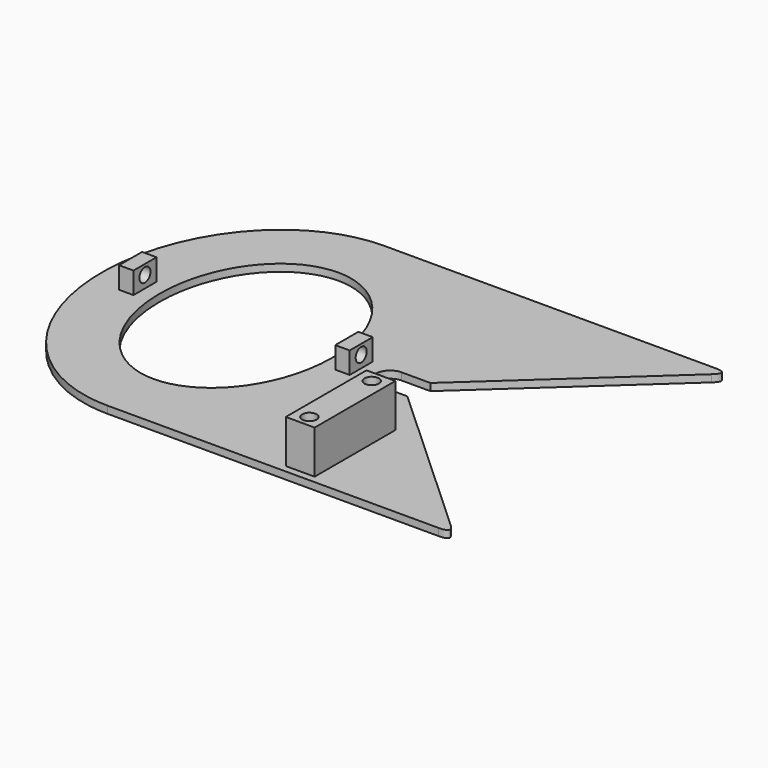
from build123d import *

# Parameters (mm, degrees)
F0_W        = 6.35
F0_H        = 12.7
F1_DEPTH    = 3.175
F3_T1_DEPTH = 35.8241837791
F4_DEPTH    = 12.7
F6_D        = 6.10108
F7_W        = 12.7
F7_H        = 44.45
F8_DEPTH    = 19.05
F9_R        = 3.175
F10_DEPTH   = 17.78
F11_DEPTH   = 17.78


# Not quite as in the source:
# - a fillet or chamfer that OpenCascade refuses, or shapes differently, is made with other operations: its cross-section is extruded or revolved along the edge and cut away or added
# - a feature of the source that left no trace in its solid (it failed there, or was rolled back) is left out


with BuildPart() as f1:
    # F0 (on Top) → F1 (new body)
    with BuildSketch(Plane.XY):
        with BuildLine():
            Line((76.2, 76.2), (-76.2, 76.2))
            add(Edge.make_bspline(
                [(-76.2, 76.2), (-139.7, 76.2), (-139.7, 0), (-139.7, -76.2), (-76.2, -76.2)],
                knots=[0, 0, 0, 1.5707963268, 1.5707963268, 3.1415926536, 3.1415926536, 3.1415926536], degree=2, weights=[1, 0.7071067812, 1, 0.7071067812, 1]))
            Line((-76.2, -76.2), (76.2, -76.2))
            Line((76.2, -76.2), (0, -6.35))
            Line((0, -6.35), (-12.7, -6.35))
            ThreePointArc((-12.7, -6.35), (-19.05, 0), (-12.7, 6.35))
            Line((-12.7, 6.35), (0, 6.35))
            Line((0, 6.35), (76.2, 76.2))
        make_face()
        with Locations((-123.825, 0)):
            Rectangle(F0_W, F0_H, mode=Mode.SUBTRACT)
        with BuildLine():
            add(Edge.make_bspline(
                [(-76.2, 50.8), (-142.1911357684, 50.8), (-109.1955678842, -25.4), (-76.2, -101.6), (-43.2044321158, -25.4), (-10.2088642316, 50.8), (-76.2, 50.8)],
                knots=[0, 0, 0, 2.0943951024, 2.0943951024, 4.1887902048, 4.1887902048, 6.2831853072, 6.2831853072, 6.2831853072], degree=2, weights=[1, 0.5, 1, 0.5, 1, 0.5, 1]))
        make_face(mode=Mode.SUBTRACT)
        with Locations((-28.575, 0)):
            Rectangle(F0_W, F0_H, mode=Mode.SUBTRACT)
    extrude(amount=F1_DEPTH)

    # F3: fillet of radius 2.54 on 2 edges, made by hand

    # F3_s2 → F3_t1 (cut)
    with BuildSketch(Plane.XY.offset(-16.3245918896)):
        with BuildLine():
            add(Edge.make_bspline(
                [(71.3865038006, 71.7876284839), (76.2, 76.2), (69.6701632442, 76.2)],
                knots=[0, 0, 0, 1, 1, 1], degree=2, weights=[1, 1, 1]))
            Line((69.6701632442, 76.2), (76.2, 76.2))
            Line((76.2, 76.2), (71.3865038006, 71.7876284839))
        make_face()
        with BuildLine():
            add(Edge.make_bspline(
                [(69.6701632442, -76.2), (76.2, -76.2), (71.3865038006, -71.7876284839)],
                knots=[0, 0, 0, 1, 1, 1], degree=2, weights=[1, 1, 1]))
            Line((71.3865038006, -71.7876284839), (76.2, -76.2))
            Line((76.2, -76.2), (69.6701632442, -76.2))
        make_face()
    extrude(amount=F3_T1_DEPTH, mode=Mode.SUBTRACT)

    # F0 (on Top) → F4 (join)
    with BuildSketch(Plane.XY):
        with Locations((-28.575, 0)):
            Rectangle(F0_W, F0_H)
        with Locations((-123.825, 0)):
            Rectangle(F0_W, F0_H)
    extrude(amount=F4_DEPTH)

    # F6 (through all)
    with Locations(Plane(origin=(-127, 0, 0), x_dir=(0, -1, 0), z_dir=(-1, 0, 0))):
        with Locations((0, 8.46836)):
            Hole(F6_D / 2)

    # F7 (on face) → F8 (join)
    with BuildSketch(Plane.XY.offset(3.175)):
        with Locations((6.1701632442, -50.8245005846)):
            Rectangle(F7_W, F7_H)
    extrude(amount=F8_DEPTH)

    # F9 (on face) → F10 (cut)
    with BuildSketch(Plane.XY.offset(22.225)):
        with Locations((6.1701632442, -67.9695005846)):
            Circle(F9_R)
    extrude(amount=-F10_DEPTH, mode=Mode.SUBTRACT)

    # F9 (on face) → F11 (cut)
    with BuildSketch(Plane.XY.offset(22.225)):
        with Locations((6.1701632442, -67.9695005846)):
            Circle(F9_R)
        with Locations((6.1701632442, -33.6795005846)):
            Circle(F9_R)
    extrude(amount=-F11_DEPTH, mode=Mode.SUBTRACT)


solid = f1.part
